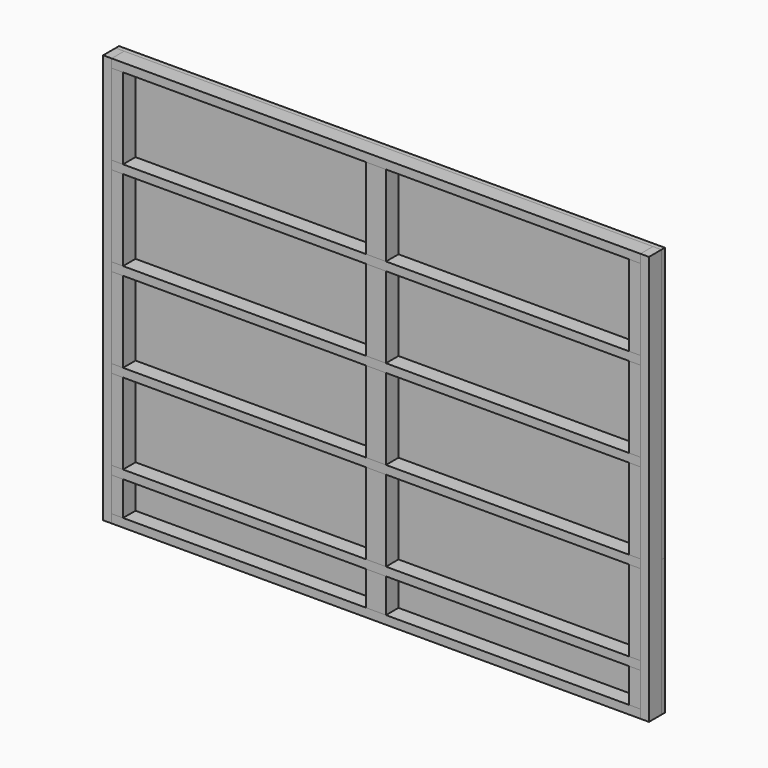
from build123d import *

# Parameters (mm, degrees)
F1_W      = 88.9
F1_H      = 1828.8
F3_DEPTH  = 88.9
F2_W      = 2362.2
F2_H      = 38.1
F4_DEPTH  = 88.9
F5_DEPTH  = 88.9
F6_DEPTH  = 88.9
F8_DEPTH  = 88.9
F7_W      = 2438.4
F7_H      = 1219.2
F7_W_2    = 2362.2
F7_H_2    = 361.95
F9_DEPTH  = 19.05
F7_H_3    = 609.6
F10_DEPTH = 19.05


# Not quite as in the source:
# - a feature names something its author has since deleted; it is built from what else it names


with BuildPart() as f3:
    # F1 (on face) → F3 (new body)
    with BuildSketch(Plane.XZ):
        with Locations((-1174.75, 0)):
            Rectangle(F1_W, F1_H)
    extrude(amount=F3_DEPTH)


with BuildPart() as f3b:
    # F1 (on face) → F3, piece 2 (new body)
    with BuildSketch(Plane.XZ):
        Rectangle(F1_W, F1_H)
    extrude(amount=F3_DEPTH)


with BuildPart() as f3c:
    # F1 (on face) → F3, piece 3 (new body)
    with BuildSketch(Plane.XZ):
        with Locations((1174.75, 0)):
            Rectangle(F1_W, F1_H)
    extrude(amount=F3_DEPTH)


with BuildPart() as f4:
    # F2 (on face) → F4 (new body)
    with BuildSketch(Plane.XZ):
        with Locations((0, 895.35)):
            Rectangle(F2_W, F2_H)
    extrude(amount=F4_DEPTH)


with BuildPart() as f4b:
    # F2 (on face) → F4, piece 2 (new body)
    with BuildSketch(Plane.XZ):
        with Locations((0, -895.35)):
            Rectangle(F2_W, F2_H)
    extrude(amount=F4_DEPTH)


with BuildPart() as f5:
    # F2 (on face) → F5 (new body)
    with BuildSketch(Plane.XZ):
        Polygon((-1181.1, 876.3), (-1181.1, 914.4), (-1219.2, 914.4), (-1219.2, -914.4), (-1181.1, -914.4), (-1181.1, -876.3), (-1181.1, -723.9), (-1181.1, -685.8), (-1181.1, -323.85), (-1181.1, -285.75), (-1181.1, 76.2), (-1181.1, 114.3), (-1181.1, 476.25), (-1181.1, 514.35), align=None)
    extrude(amount=F5_DEPTH)


with BuildPart() as f5b:
    # F2 (on face) → F5, piece 2 (new body)
    with BuildSketch(Plane.XZ):
        Polygon((1219.2, 914.4), (1181.1, 914.4), (1181.1, 876.3), (1181.1, 514.35), (1181.1, 476.25), (1181.1, 114.3), (1181.1, 76.2), (1181.1, -285.75), (1181.1, -323.85), (1181.1, -685.8), (1181.1, -723.9), (1181.1, -876.3), (1181.1, -914.4), (1219.2, -914.4), align=None)
    extrude(amount=F5_DEPTH)


with BuildPart() as f6:
    # F2 (on face) → F6 (new body)
    with BuildSketch(Plane.XZ):
        with Locations((0, 495.3)):
            Rectangle(F2_W, F2_H)
    extrude(amount=F6_DEPTH)


with BuildPart() as f6b:
    # F2 (on face) → F6, piece 2 (new body)
    with BuildSketch(Plane.XZ):
        with Locations((0, 95.25)):
            Rectangle(F2_W, F2_H)
    extrude(amount=F6_DEPTH)


with BuildPart() as f6c:
    # F2 (on face) → F6, piece 3 (new body)
    with BuildSketch(Plane.XZ):
        with Locations((0, -304.8)):
            Rectangle(F2_W, F2_H)
    extrude(amount=F6_DEPTH)


with BuildPart() as f8:
    # F2 (on face) → F8 (new body)
    with BuildSketch(Plane.XZ):
        with Locations((0, -304.8)):
            Rectangle(F2_W, F2_H)
    extrude(amount=F8_DEPTH)


with BuildPart() as f8b:
    # F2 (on face) → F8, piece 2 (new body)
    with BuildSketch(Plane.XZ):
        with Locations((0, -704.85)):
            Rectangle(F2_W, F2_H)
    extrude(amount=F8_DEPTH)


with BuildPart() as f9:
    # F7 (on face) → F9 (new body)
    with BuildSketch(Plane.XZ):
        with Locations((0, 304.8)):
            Rectangle(F7_W, F7_H)
        with Locations((0, 295.275)):
            Rectangle(F7_W_2, F7_H_2, mode=Mode.SUBTRACT)
        with Locations((0, 295.275)):
            Rectangle(F7_W_2, F7_H_2)
    extrude(amount=F9_DEPTH)


with BuildPart() as f10:
    # F7 (on face) → F10 (new body)
    with BuildSketch(Plane.XZ):
        with Locations((0, -609.6)):
            Rectangle(F7_W, F7_H_3)
    extrude(amount=F10_DEPTH)


solid = Compound([f3.part, f3b.part, f3c.part, f4.part, f4b.part, f5.part, f5b.part, f6.part, f6b.part, f6c.part, f8.part, f8b.part, f9.part, f10.part])
